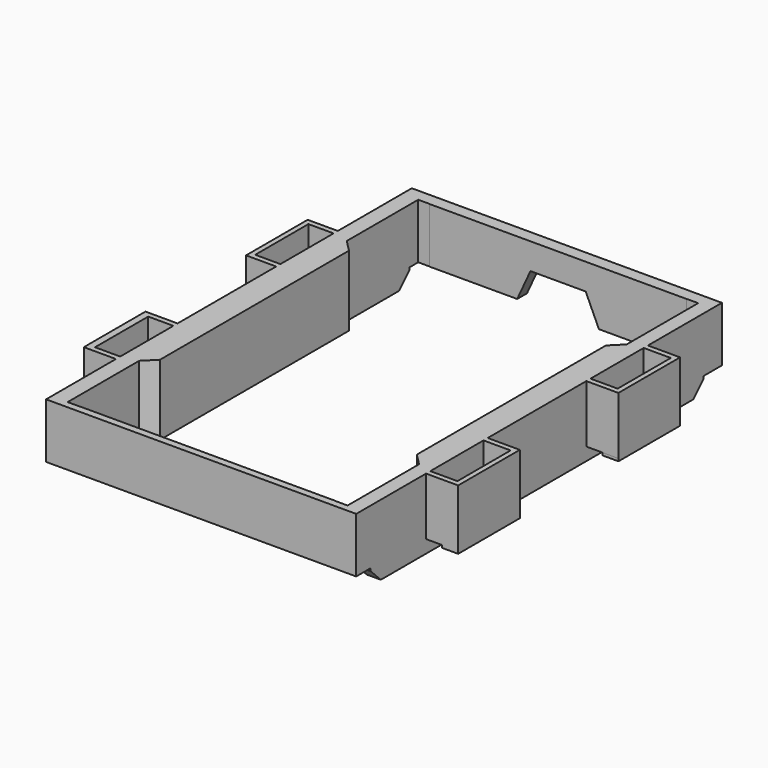
from build123d import *

# Parameters (mm, degrees)
F0_W          = 60.96
F0_H          = 91.44
F0_W_2        = 50.8
F0_H_2        = 86.614
F1_DEPTH      = 28.448
F3_DEPTH      = 25.4
F4_W          = 66.649839282
F4_H          = 6.9823637605
F5_DEPTH      = 3.048
F6_W          = 64.9686481762
F6_H          = 4.777956934
F7_DEPTH      = 3.048
F9_DEPTH      = 2.286
F10_W         = 99.848318845
F10_H         = 48.2080141082
F11_DEPTH     = 50.8
F13_T1_DEPTH  = 15.8581495789
F13_T3_DEPTH  = 15.8581495789
F13_T8_DEPTH  = 41.5121495789
F13_T13_DEPTH = 41.5121495789
F13_T18_DEPTH = 41.5121495789
F13_T23_DEPTH = 41.5121495789
F14_W         = 15.24
F14_H         = 23.368
F15_DEPTH     = 6.35
F16_W         = 5.3607832682
F16_H         = 13.1506472826
F17_DEPTH     = 25.909
F19_DEPTH     = 0.254
F20_DEPTH     = 0.254
F21_DEPTH     = 1.016
F22_W         = 3.175
F22_H         = 15.24
F22_H_2       = 15.425526537
F23_DEPTH     = 0.508
F24_W         = 3.175
F24_H         = 15.24
F24_H_2       = 15.1729788631
F25_DEPTH     = 0.508
F26_W         = 1.4869117904
F26_H         = 15.24
F26_H_2       = 15.1544166729
F27_DEPTH     = 0.508
F28_W         = 1.5113
F28_H         = 15.24
F28_W_2       = 1.492887156
F28_H_2       = 15.3870563954
F29_DEPTH     = 0.254
F30_DEPTH     = 0.381
F31_DEPTH     = 0.254
F32_W         = 105.9566885233
F32_H         = 116.2753328681
F33_DEPTH     = 14.5


# Not quite as in the source:
# - a fillet or chamfer that OpenCascade refuses, or shapes differently, is made with other operations: its cross-section is extruded or revolved along the edge and cut away or added
# - a feature names something its author has since deleted; it is built from what else it names


with BuildPart() as f1:
    # F0 (on Top) → F1 (new body)
    with BuildSketch(Plane.XY):
        Rectangle(F0_W, F0_H)
        Rectangle(F0_W_2, F0_H_2, mode=Mode.SUBTRACT)
    extrude(amount=F1_DEPTH)

    # F2 (on face) → F3 (cut)
    with BuildSketch(Plane(origin=(0, 45.72, 0), x_dir=(-1, 0, 0), z_dir=(0, 1, 0))):
        Polygon((-9.4803553075, 0), (0, 0), (9.4803553075, 0), (5.461, 8.763), (-5.461, 8.763), align=None)
        Polygon((-9.4803553075, 28.448), (-5.461, 19.685), (5.461, 19.685), (9.4803553075, 28.448), (0, 28.448), align=None)
    extrude(amount=-F3_DEPTH, mode=Mode.SUBTRACT)

    # F4 (on Top) → F5 (cut)
    with BuildSketch(Plane.XY):
        with Locations((-0.1057945192, 44.6448102593)):
            Rectangle(F4_W, F4_H)
        with Locations((-0.1057945192, -44.6448102593)):
            Rectangle(F4_W, F4_H)
    extrude(amount=F5_DEPTH, mode=Mode.SUBTRACT)

    # F6 (on face) → F7 (cut)
    with BuildSketch(Plane.XY.offset(28.448)):
        with Locations((-2.0043240881, 43.331021533)):
            Rectangle(F6_W, F6_H)
        with Locations((-2.0043240881, -43.331021533)):
            Rectangle(F6_W, F6_H)
    extrude(amount=-F7_DEPTH, mode=Mode.SUBTRACT)

    # F8 (on face) → F9 (cut)
    with BuildSketch(Plane(origin=(25.4, 0, 0), x_dir=(0, -1, 0), z_dir=(-1, 0, 0))):
        Polygon((-43.0863499641, 0), (-41.1536283791, 0), (-25.9136283791, 0), (-25.9136283791, 30.48), (-41.1536283791, 30.48), (-43.0863499641, 30.48), align=None)
        Polygon((25.9136283791, 30.48), (25.9136283791, 0), (41.1536283791, 0), (43.0863499641, 0), (43.0863499641, 30.48), (41.1536283791, 30.48), align=None)
    extrude(amount=-F9_DEPTH, mode=Mode.SUBTRACT)

    # F10 (on Right) → F11 (cut)
    with BuildSketch(Plane.YZ):
        with Locations((1.7518345267, 13.4315635078)):
            Rectangle(F10_W, F10_H)
    extrude(amount=-F11_DEPTH, mode=Mode.SUBTRACT)

    # F12: F1 across plane


with BuildPart() as f1_1:
    add(f1.part)
    add(f1.part.mirror(Plane.YZ))

    # F13: chamfer of 2.54 on 12 edges, made by hand

    # F13_s2 → F13_t1 (cut)
    with BuildSketch(Plane.YZ.offset(-37.0120747894)):
        Polygon((38.402043066, 28.448), (40.942043066, 25.908), (40.942043066, 28.448), align=None)
        Polygon((38.6136283791, 0), (41.1536283791, 2.54), (41.1536283791, 0), align=None)
        Polygon((-40.942043066, 25.908), (-38.402043066, 28.448), (-40.942043066, 28.448), align=None)
        Polygon((-38.6136283791, 0), (-41.1536283791, 2.54), (-41.1536283791, 0), align=None)
    extrude(amount=F13_T1_DEPTH, mode=Mode.SUBTRACT)

    # F13_s4 → F13_t3 (cut)
    with BuildSketch(Plane.YZ.offset(21.1539252106)):
        Polygon((38.402043066, 28.448), (40.942043066, 25.908), (40.942043066, 28.448), align=None)
        Polygon((-40.942043066, 25.908), (-38.402043066, 28.448), (-40.942043066, 28.448), align=None)
        Polygon((-38.6136283791, 0), (-41.1536283791, 2.54), (-41.1536283791, 0), align=None)
        Polygon((38.6136283791, 0), (41.1536283791, 2.54), (41.1536283791, 0), align=None)
    extrude(amount=F13_T3_DEPTH, mode=Mode.SUBTRACT)


with BuildPart() as f13_tool6:
    # F13_s7 → F13_t8 (new body)
    with BuildSketch(Plane.XY.offset(-6.5320747894)):
        Polygon((25.4, 23.3736283791), (27.94, 25.9136283791), (25.4, 25.9136283791), align=None)
    extrude(amount=F13_T8_DEPTH)

    split(bisect_by=Plane.YZ.offset(27.686), keep=Keep.BOTTOM)


with BuildPart() as f1_2:
    add(f1_1.part)

    # F13_t5: cut F13_tool6
    add(f13_tool6.part, mode=Mode.SUBTRACT)


with BuildPart() as f13_tool11:
    # F13_s12 → F13_t13 (new body)
    with BuildSketch(Plane.XY.offset(34.9800747894)):
        Polygon((25.4, -23.3736283791), (27.94, -25.9136283791), (25.4, -25.9136283791), align=None)
    extrude(amount=-F13_T13_DEPTH)

    split(bisect_by=Plane.YZ.offset(27.686), keep=Keep.BOTTOM)


with BuildPart() as f1_3:
    add(f1_2.part)

    # F13_t10: cut F13_tool11
    add(f13_tool11.part, mode=Mode.SUBTRACT)


with BuildPart() as f13_tool16:
    # F13_s17 → F13_t18 (new body)
    with BuildSketch(Plane.XY.offset(-6.5320747894)):
        Polygon((-27.94, 25.9136283791), (-25.4, 23.3736283791), (-25.4, 25.9136283791), align=None)
    extrude(amount=F13_T18_DEPTH)

    split(bisect_by=Plane.YZ.offset(-27.686), keep=Keep.TOP)


with BuildPart() as f1_4:
    add(f1_3.part)

    # F13_t15: cut F13_tool16
    add(f13_tool16.part, mode=Mode.SUBTRACT)


with BuildPart() as f13_tool21:
    # F13_s22 → F13_t23 (new body)
    with BuildSketch(Plane.XY.offset(34.9800747894)):
        Polygon((-25.4, -23.3736283791), (-27.94, -25.9136283791), (-25.4, -25.9136283791), align=None)
    extrude(amount=-F13_T23_DEPTH)

    split(bisect_by=Plane.YZ.offset(-27.686), keep=Keep.TOP)


with BuildPart() as f1_5:
    add(f1_4.part)

    # F13_t20: cut F13_tool21
    add(f13_tool21.part, mode=Mode.SUBTRACT)

    # F14 (on face) → F15 (join)
    with BuildSketch(Plane.YZ.offset(30.48)):
        with Locations((-19.812, 14.224)):
            Rectangle(F14_W, F14_H)
        with Locations((19.812, 14.224)):
            Rectangle(F14_W, F14_H)
    extrude(amount=F15_DEPTH)

    # F16 (on face) → F17 (cut, through all)
    with BuildSketch(Plane.XY.offset(25.908)):
        with Locations((33.1603916341, -19.8066011071)):
            Rectangle(F16_W, F16_H)
        with Locations((33.1603916341, 19.8066011071)):
            Rectangle(F16_W, F16_H)
    extrude(amount=-F17_DEPTH, mode=Mode.SUBTRACT)

    # F18: F1 across plane


with BuildPart() as f1_6:
    add(f1_5.part)
    add(f1_5.part.mirror(Plane.YZ))

    # F19 (cut): faces of the model
    f19_faces = [f1_6.faces().sort_by_distance(p)[0] for p in [
        (26.543, -43.0863499641, 14.224),
        (-26.543, -43.0863499641, 14.224),
    ]]
    extrude(f19_faces, amount=-F19_DEPTH, mode=Mode.SUBTRACT)

    # F20 (cut): faces of the model
    f20_faces = [f1_6.faces().sort_by_distance(p)[0] for p in [
        (26.543, 43.0863499641, 14.224),
        (-26.543, 43.0863499641, 14.224),
    ]]
    extrude(f20_faces, amount=-F20_DEPTH, mode=Mode.SUBTRACT)

    # F21 (cut): a face of the model
    f21_faces = [f1_6.faces().sort_by_distance(p)[0] for p in [
        (0, -45.72, 14.224),
    ]]
    extrude(f21_faces, amount=-F21_DEPTH, mode=Mode.SUBTRACT)

    # F22 (on face) → F23 (join)
    with BuildSketch(Plane.XY.offset(25.908)):
        with Locations((-35.2425, 19.812)):
            Rectangle(F22_W, F22_H)
        with Locations((-35.2425, -19.7230628692)):
            Rectangle(F22_W, F22_H_2)
    extrude(amount=F23_DEPTH)

    # F24 (on face) → F25 (join)
    with BuildSketch(Plane(origin=(0, 0, 2.54), x_dir=(1, 0, 0), z_dir=(0, 0, -1))):
        with Locations((35.2425, 19.812)):
            Rectangle(F24_W, F24_H)
        with Locations((35.2425, -19.7903430089)):
            Rectangle(F24_W, F24_H_2)
    extrude(amount=F25_DEPTH)

    # F26 (on face) → F27 (join)
    with BuildSketch(Plane.XY.offset(25.908)):
        with Locations((36.0865441048, -19.812)):
            Rectangle(F26_W, F26_H)
        with Locations((36.0865441048, 19.7994005866)):
            Rectangle(F26_W, F26_H_2)
    extrude(amount=F27_DEPTH)

    # F28 (on face) → F29 (join)
    with BuildSketch(Plane(origin=(0, 0, 2.54), x_dir=(1, 0, 0), z_dir=(0, 0, -1))):
        with Locations((-36.07435, 19.812)):
            Rectangle(F28_W, F28_H)
        with Locations((-36.083556422, -19.7531366721)):
            Rectangle(F28_W_2, F28_H_2)
    extrude(amount=F29_DEPTH)

    # F30 (add): faces of the model
    f30_faces = [f1_6.faces().sort_by_distance(p)[0] for p in [
        (-30.48, 0.4258489378, 14.2172059936),
        (-35.3187, -19.812, 2.413),
        (-35.8407832682, -19.8066011071, 14.224),
        (-36.83, -19.8101053315, 14.3540262363),
    ]]
    extrude(f30_faces, amount=F30_DEPTH, dir=(-1, 0, 0))

    # F31 (add): a face of the model
    f31_faces = [f1_6.faces().sort_by_distance(p)[0] for p in [
        (-35.337112844, 19.7531366721, 2.413),
    ]]
    extrude(f31_faces, amount=F31_DEPTH)

    # F32 (on face) → F33 (cut)
    with BuildSketch(Plane.XY.offset(28.448)):
        with Locations((11.0789313912, -7.9427920282)):
            Rectangle(F32_W, F32_H)
    extrude(amount=-F33_DEPTH, mode=Mode.SUBTRACT)


solid = f1_6.part
